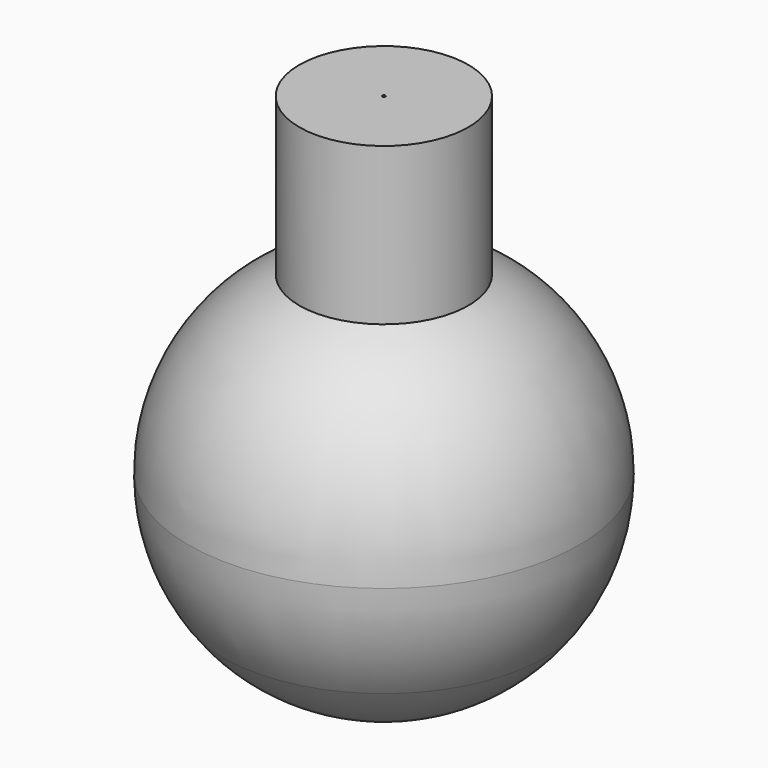
from build123d import *


# Not quite as in the source:
# - ends of sketch curves that miss each other by under 0.0002 mm in the source are joined
# - a feature names something its author has since deleted; it is built from what else it names


with BuildPart() as f1:
    # F0 (on Front) → F1 (revolve)
    with BuildSketch(Plane.XZ):
        with BuildLine():
            Line((-124.4340789334, 127), (0, 127))
            Line((0, 127), (0, 177.8))
            ThreePointArc((0, 177.8), (-39.0537400688, 173.4579066709), (-76.2, 160.6437051366))
            ThreePointArc((-76.2, 160.6437051366), (-101.7176317641, 145.8299125293), (-124.4340789334, 127))
        make_face()
        with BuildLine():
            Line((-177.8, 0), (0, 0))
            Line((0, 0), (0, 127))
            Line((0, 127), (-124.4340789334, 127))
            ThreePointArc((-124.4340789334, 127), (-163.9164563275, 68.8784098615), (-177.8, 0))
        make_face()
        with BuildLine():
            Line((1.4081087779, -101.6), (0, 0))
            Line((0, 0), (-177.8, 0))
            ThreePointArc((-177.8, 0), (-169.6407590458, -53.2433363939), (-145.9118912221, -101.6))
            Line((-145.9118912221, -101.6), (1.4081087779, -101.6))
        make_face()
        with BuildLine():
            Line((1.4081087779, -165.1), (1.4081087779, -101.6))
            Line((1.4081087779, -101.6), (-145.9118912221, -101.6))
            ThreePointArc((-145.9118912221, -101.6), (-110.4662750061, -139.3199270969), (-65.6586544962, -165.2325061534))
            Line((-65.6586544962, -165.2325061534), (1.4081087779, -165.1))
        make_face()
        with BuildLine():
            ThreePointArc((-76.2, 160.6437051366), (-39.0537400688, 173.4579066709), (0, 177.8))
            Line((0, 177.8), (0, 304.8))
            Line((0, 304.8), (-76.2, 304.8))
            Line((-76.2, 304.8), (-76.2, 160.6437051366))
        make_face()
    revolve(axis=Axis((1.4081087779, 0, -133.35), (0, 0, 1)))


solid = f1.part
